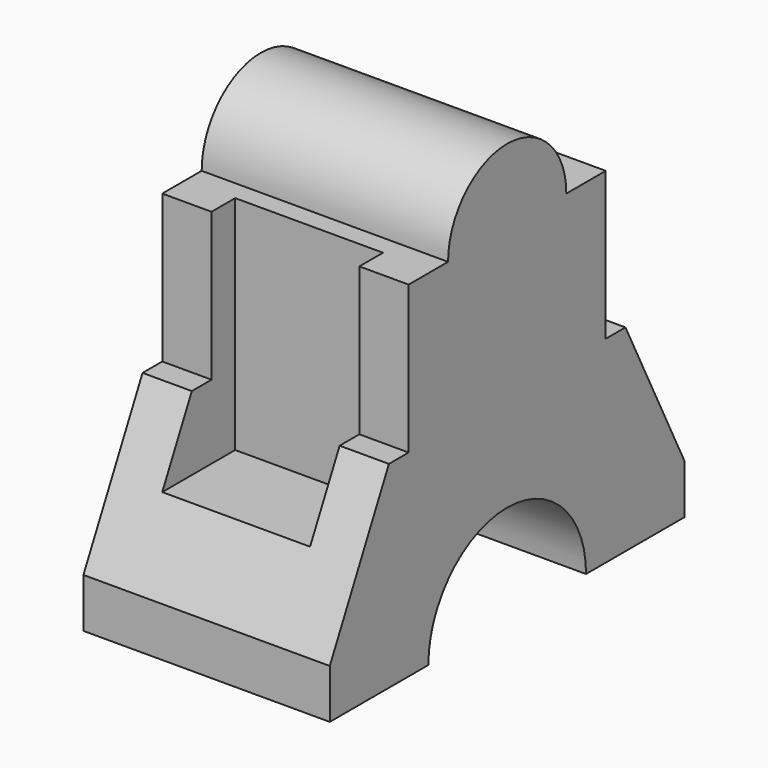
from build123d import *

# Parameters (mm, degrees)
F1_DEPTH = 25
F2_R     = 20
F3_DEPTH = 50.001
F4_R     = 15
F5_DEPTH = 50
F6_W     = 30
F6_H     = 45
F7_DEPTH = 26


# Not quite as in the source:
# - a pattern or mirror of a feature is missing from the dataset's text; its kind, count and spacing are read off the source's solid


with BuildPart() as f1:
    # F0 (on Right) → F1 (new body, symmetric)
    with BuildSketch(Plane.YZ):
        Polygon((-45, 0), (0, 0), (45, 0), (45, 10), (30, 40), (25, 40), (25, 70), (0, 70), (-25, 70), (-25, 40), (-30, 40), (-45, 10), align=None)
    extrude(amount=F1_DEPTH, both=True)

    # F2 (on face) → F3 (cut, through all)
    with BuildSketch(Plane.YZ.offset(25)):
        Circle(F2_R)
    extrude(amount=-F3_DEPTH, mode=Mode.SUBTRACT)

    # F4 (on face) → F5 (join)
    with BuildSketch(Plane.YZ.offset(25)):
        with Locations((0, 70)):
            Circle(F4_R)
    extrude(amount=-F5_DEPTH)

    # F6 (on face) → F7 (cut)
    with BuildSketch(Plane.XZ.offset(45)):
        with Locations((0, 47.5)):
            Rectangle(F6_W, F6_H)
    f7 = extrude(amount=-F7_DEPTH, mode=Mode.SUBTRACT)

    # F7_copies: F7 across plane
    add(f7.mirror(Plane.ZX), mode=Mode.SUBTRACT)


solid = f1.part
